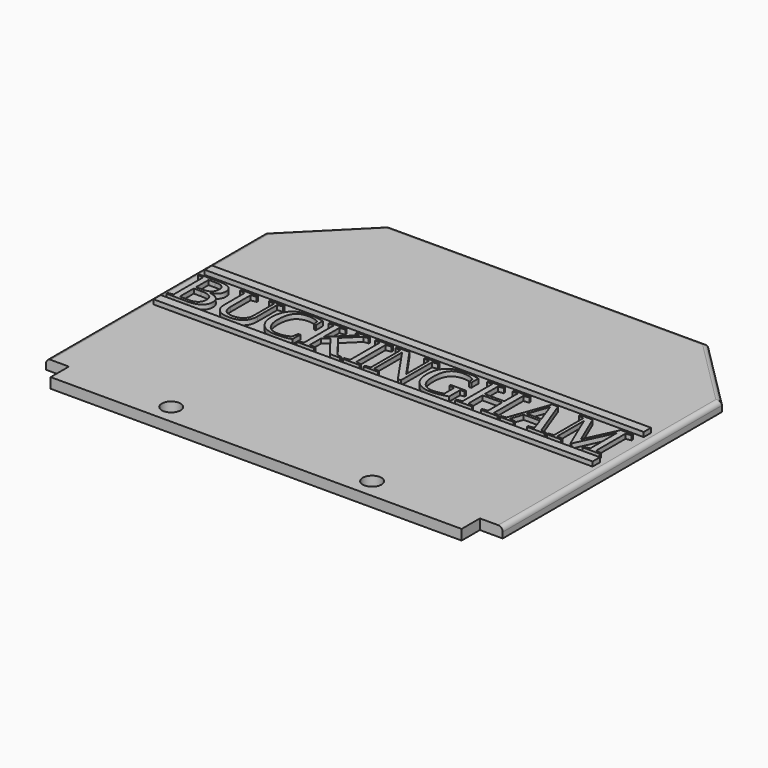
from build123d import *

# Parameters (mm, degrees)
F0_R         = 2.05
F1_DEPTH     = 2.25
F2_W         = 96.1458333333
F2_H         = 2
F2_TEXT_SIZE = 13.8888888889
F3_DEPTH     = 1
F4_SIZE      = 15
F5_R         = 1


# Not quite as in the source:
# - Text() gives the source's letters only with a copy of the font that has no kerning and outlines rounded to 1/6400 em; it was checked with that copy


with BuildPart() as f1:
    # F0 (on Top) → F1 (new body)
    with BuildSketch(Plane.XY):
        Polygon((-45, -35), (-45, -40), (45, -40), (45, -35), (50, -35), (50, 40), (-50, 40), (-50, -35), align=None)
        with Locations((-22, -35.75)):
            Circle(F0_R, mode=Mode.SUBTRACT)
        with Locations((22, -35.75)):
            Circle(F0_R, mode=Mode.SUBTRACT)
    extrude(amount=F1_DEPTH)

    # F2 (on face) → F3 (join)
    with BuildSketch(Plane.XY.offset(2.25)):
        with Locations((-8.33333e-05, -6.9999999995)):
            Rectangle(F2_W, F2_H)
        Polygon((-48.0728095102, 8.0011445925), (-48.0728571292, 6.001144593), (48.0729761769, 5.9988554065), (48.0730237959, 7.998855406), align=None)
        with Locations((-48.073, -5)):
            Text('BUCKINGHAM', F2_TEXT_SIZE, font='Tinos', text_align=(TextAlign.LEFT, TextAlign.BOTTOM))
    extrude(amount=F3_DEPTH)

    # F4
    f4_edges = [f1.edges().sort_by_distance(p)[0] for p in [
        (-50, 40, 1.125),
        (50, 40, 1.125),
    ]]
    chamfer(f4_edges, length=F4_SIZE)

    # F5
    f5_edges = [f1.edges().sort_by_distance(p)[0] for p in [
        (0, 40, 2.25),
        (-42.5, 32.5, 2.25),
        (-50, -5, 2.25),
        (42.5, 32.5, 2.25),
        (50, -5, 2.25),
    ]]
    fillet(f5_edges, radius=F5_R)


solid = f1.part
